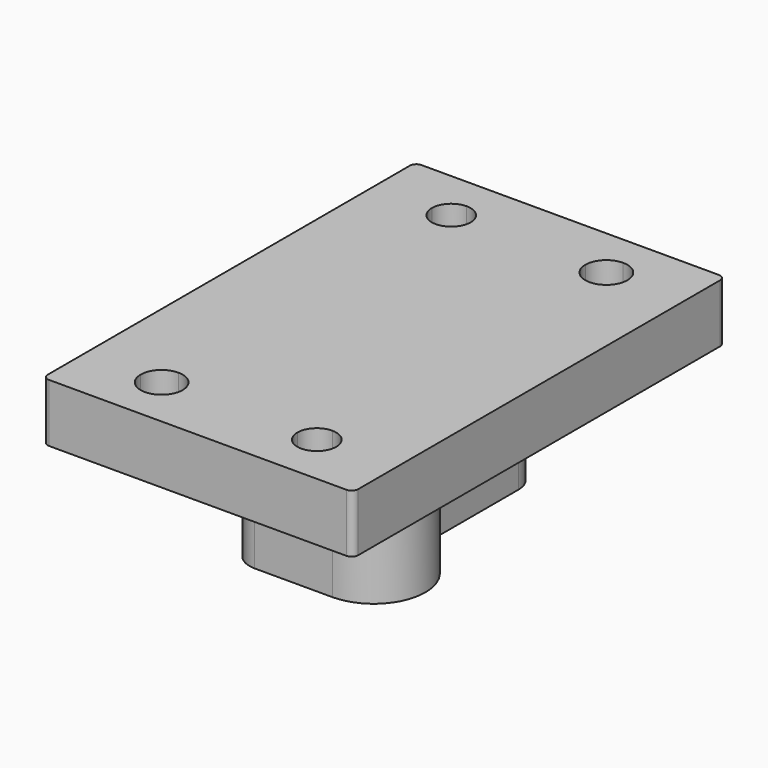
from build123d import *

# Parameters (mm, degrees)
F1_DEPTH = 41.275
F3_DEPTH = 14.2875
F5_DEPTH = 14.2875


with BuildPart() as f1:
    # F0 (on Top) → F1 (new body)
    with BuildSketch(Plane.XY):
        with BuildLine():
            Line((-6.3457395977, -31.7500010133), (12.7042604023, -31.7500010133))
            ThreePointArc((12.7042604023, -31.7500010133), (25.4042604023, -19.0500010133), (12.7042604023, -6.3500010133))
            Line((12.7042604023, -6.3500010133), (12.7042604023, 25.3999989867))
            ThreePointArc((12.7042604023, 25.3999989867), (10.8443884629, 29.8901270473), (6.3542604023, 31.7499989867))
            Line((6.3542604023, 31.7499989867), (-12.6957395977, 31.7499989867))
            ThreePointArc((-12.6957395977, 31.7499989867), (-25.3957395977, 19.0499989867), (-12.6957395977, 6.3499989867))
            Line((-12.6957395977, 6.3499989867), (-12.6957395977, -25.4000010133))
            ThreePointArc((-12.6957395977, -25.4000010133), (-10.8358676582, -29.8901290738), (-6.3457395977, -31.7500010133))
        make_face()
    extrude(amount=-F1_DEPTH)

    # F2 (on face) → F3 (join)
    with BuildSketch(Plane.XY):
        with BuildLine():
            Line((-36.5125, -57.15), (36.5125, -57.15))
            ThreePointArc((36.5125, -57.15), (37.6350320151, -56.6850320151), (38.1, -55.5625))
            Line((38.1, -55.5625), (38.1, 55.5625))
            ThreePointArc((38.1, 55.5625), (37.6350320151, 56.6850320151), (36.5125, 57.15))
            Line((36.5125, 57.15), (-36.5125, 57.15))
            ThreePointArc((-36.5125, 57.15), (-37.6350320151, 56.6850320151), (-38.1, 55.5625))
            Line((-38.1, 55.5625), (-38.1, -55.5625))
            ThreePointArc((-38.1, -55.5625), (-37.6350320151, -56.6850320151), (-36.5125, -57.15))
        make_face()
        with BuildLine():
            Line((-12.6957395977, 31.7499989867), (6.3542604023, 31.7499989867))
            ThreePointArc((6.3542604023, 31.7499989867), (10.8443884629, 29.8901270473), (12.7042604023, 25.3999989867))
            Line((12.7042604023, 25.3999989867), (12.7042604023, -6.3500010133))
            ThreePointArc((12.7042604023, -6.3500010133), (25.4042604023, -19.0500010133), (12.7042604023, -31.7500010133))
            Line((12.7042604023, -31.7500010133), (-6.3457395977, -31.7500010133))
            ThreePointArc((-6.3457395977, -31.7500010133), (-10.8358676582, -29.8901290738), (-12.6957395977, -25.4000010133))
            Line((-12.6957395977, -25.4000010133), (-12.6957395977, 6.3499989867))
            ThreePointArc((-12.6957395977, 6.3499989867), (-25.3957395977, 19.0499989867), (-12.6957395977, 31.7499989867))
        make_face(mode=Mode.SUBTRACT)
    extrude(amount=-F3_DEPTH)

    # F4 (on face) → F5 (cut)
    with BuildSketch(Plane.XY):
        with BuildLine():
            Line((19.05, 39.2938), (19.05, 44.45))
            Line((19.05, 44.45), (13.8938, 44.45))
            ThreePointArc((13.8938, 44.45), (15.4040160148, 40.8040160148), (19.05, 39.2938))
        make_face()
        with BuildLine():
            Line((19.05, 44.45), (24.2062, 44.45))
            ThreePointArc((24.2062, 44.45), (22.6959839852, 48.0959839852), (19.05, 49.6062))
            Line((19.05, 49.6062), (19.05, 44.45))
        make_face()
        with BuildLine():
            Line((19.05, 44.45), (19.05, 49.6062))
            ThreePointArc((19.05, 49.6062), (15.4040160148, 48.0959839852), (13.8938, 44.45))
            Line((13.8938, 44.45), (19.05, 44.45))
        make_face()
        with BuildLine():
            ThreePointArc((19.05, 39.2938), (22.6959839852, 40.8040160148), (24.2062, 44.45))
            Line((24.2062, 44.45), (19.05, 44.45))
            Line((19.05, 44.45), (19.05, 39.2938))
        make_face()
        with BuildLine():
            Line((-19.05, -44.45), (-13.8938, -44.45))
            ThreePointArc((-13.8938, -44.45), (-15.4040160148, -40.8040160148), (-19.05, -39.2938))
            Line((-19.05, -39.2938), (-19.05, -44.45))
        make_face()
        with BuildLine():
            ThreePointArc((-19.05, -49.6062), (-15.4040160148, -48.0959839852), (-13.8938, -44.45))
            Line((-13.8938, -44.45), (-19.05, -44.45))
            Line((-19.05, -44.45), (-19.05, -49.6062))
        make_face()
        with BuildLine():
            ThreePointArc((-24.2062, -44.45), (-22.6959839852, -48.0959839852), (-19.05, -49.6062))
            Line((-19.05, -49.6062), (-19.05, -44.45))
            Line((-19.05, -44.45), (-24.2062, -44.45))
        make_face()
        with BuildLine():
            Line((-24.2062, -44.45), (-19.05, -44.45))
            Line((-19.05, -44.45), (-19.05, -39.2938))
            ThreePointArc((-19.05, -39.2938), (-22.6959839852, -40.8040160148), (-24.2062, -44.45))
        make_face()
        with BuildLine():
            Line((-14.2875, 44.45), (-19.05, 44.45))
            Line((-19.05, 44.45), (-19.05, 39.6875))
            ThreePointArc((-19.05, 39.6875), (-15.6824039546, 41.0824039546), (-14.2875, 44.45))
        make_face()
        with BuildLine():
            ThreePointArc((-14.2875, 44.45), (-15.6824039546, 47.8175960454), (-19.05, 49.2125))
            Line((-19.05, 49.2125), (-19.05, 44.45))
            Line((-19.05, 44.45), (-14.2875, 44.45))
        make_face()
        with BuildLine():
            Line((-19.05, 44.45), (-19.05, 49.2125))
            ThreePointArc((-19.05, 49.2125), (-22.4175960454, 47.8175960454), (-23.8125, 44.45))
            Line((-23.8125, 44.45), (-19.05, 44.45))
        make_face()
        with BuildLine():
            Line((-19.05, 39.6875), (-19.05, 44.45))
            Line((-19.05, 44.45), (-23.8125, 44.45))
            ThreePointArc((-23.8125, 44.45), (-22.4175960454, 41.0824039546), (-19.05, 39.6875))
        make_face()
        with BuildLine():
            Line((19.05, -44.45), (23.8125, -44.45))
            ThreePointArc((23.8125, -44.45), (22.4175960454, -41.0824039546), (19.05, -39.6875))
            Line((19.05, -39.6875), (19.05, -44.45))
        make_face()
        with BuildLine():
            Line((14.2875, -44.45), (19.05, -44.45))
            Line((19.05, -44.45), (19.05, -39.6875))
            ThreePointArc((19.05, -39.6875), (15.6824039546, -41.0824039546), (14.2875, -44.45))
        make_face()
        with BuildLine():
            Line((19.05, -49.2125), (19.05, -44.45))
            Line((19.05, -44.45), (14.2875, -44.45))
            ThreePointArc((14.2875, -44.45), (15.6824039546, -47.8175960454), (19.05, -49.2125))
        make_face()
        with BuildLine():
            ThreePointArc((19.05, -49.2125), (22.4175960454, -47.8175960454), (23.8125, -44.45))
            Line((23.8125, -44.45), (19.05, -44.45))
            Line((19.05, -44.45), (19.05, -49.2125))
        make_face()
    extrude(amount=-F5_DEPTH, mode=Mode.SUBTRACT)


solid = f1.part
